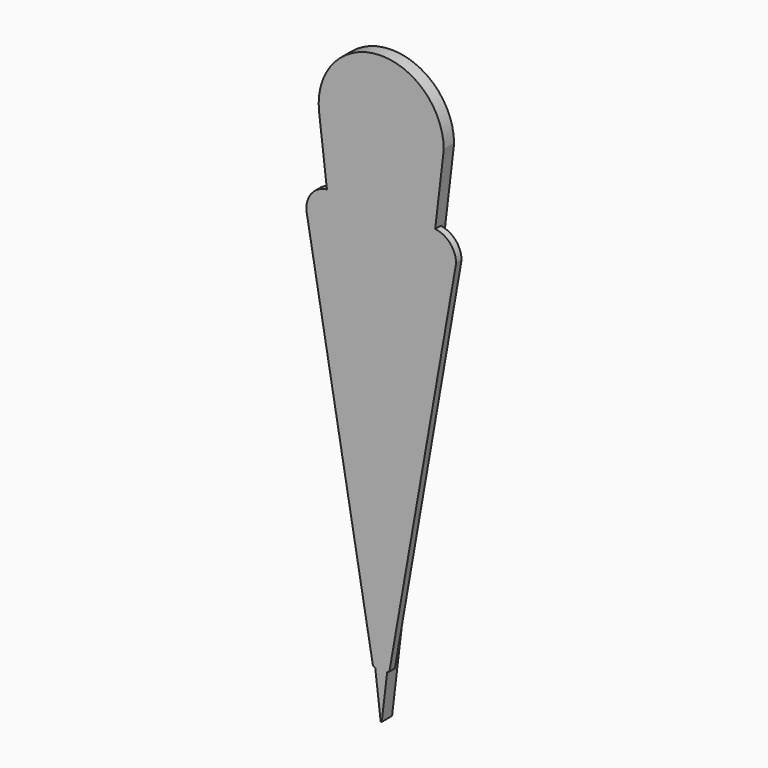
from build123d import *

# Parameters (mm, degrees)
F1_DEPTH = 1.778
F2_DEPTH = 1.5748
F3_DEPTH = 1.778


with BuildPart() as f1:
    # F0 (on Front) → F1 (new body)
    with BuildSketch(Plane.XZ):
        with BuildLine():
            Line((14.02935353, 41.1213250894), (16.2583384663, 59.9522180855))
            ThreePointArc((16.2583384663, 59.9522180855), (-0.9637356423, 76.1819680311), (-16.1440849231, 58.0281360497))
            Line((-16.1440849231, 58.0281360497), (-14.1149313353, 41.0024441959))
            Line((-14.1149313353, 41.0024441959), (-1.6278814086, -63.7706323678))
            Line((-1.6278814086, -63.7706323678), (-1.5574045531, -64.3619711562))
            Line((-1.5574045531, -64.3619711562), (-0.1437664474, -76.223156493))
            ThreePointArc((-0.1437664474, -76.223156493), (-0.0022464, -76.237388177), (0.1393582085, -76.2240240658))
            Line((0.1393582085, -76.2240240658), (1.5482228022, -64.3216652936))
            Line((1.5482228022, -64.3216652936), (14.02935353, 41.1213250894))
        make_face()
    extrude(amount=F1_DEPTH)

    # F2 (add): a face of the model
    f2_faces = [f1.faces().sort_by_distance(p)[0] for p in [
        (-0.03237785, 0, 22.4036287073),
    ]]
    extrude(f2_faces, amount=F2_DEPTH)

    # F0 (on Front) → F3 (join)
    with BuildSketch(Plane.XZ):
        with BuildLine():
            ThreePointArc((19.465577211, 35.0036723741), (17.9101589408, 39.0956829635), (14.02935353, 41.1213250894))
            Line((14.02935353, 41.1213250894), (1.5482228022, -64.3216652936))
            ThreePointArc((1.5482228022, -64.3216652936), (1.9456415345, -64.2155103566), (2.1613873882, -63.865275798))
            ThreePointArc((2.1613873882, -63.865275798), (2.1676286256, -63.8175184176), (2.1697142526, -63.7694001198))
            Line((2.1697142526, -63.7694001198), (2.1781676915, -63.7694001198))
            Line((2.1781676915, -63.7694001198), (19.465577211, 35.0036723741))
        make_face()
        with BuildLine():
            Line((-1.6278814086, -63.7706323678), (-14.1149313353, 41.0024441959))
            ThreePointArc((-14.1149313353, 41.0024441959), (-18.2559821933, 38.6033472019), (-19.3598979472, 33.9465952648))
            Line((-19.3598979472, 33.9465952648), (-2.2124765092, -63.7709956311))
            ThreePointArc((-2.2124765092, -63.7709956311), (-2.0162187298, -64.2119998537), (-1.5574045531, -64.3619711562))
            Line((-1.5574045531, -64.3619711562), (-1.6278814086, -63.7706323678))
        make_face()
    extrude(amount=F3_DEPTH)


solid = f1.part
